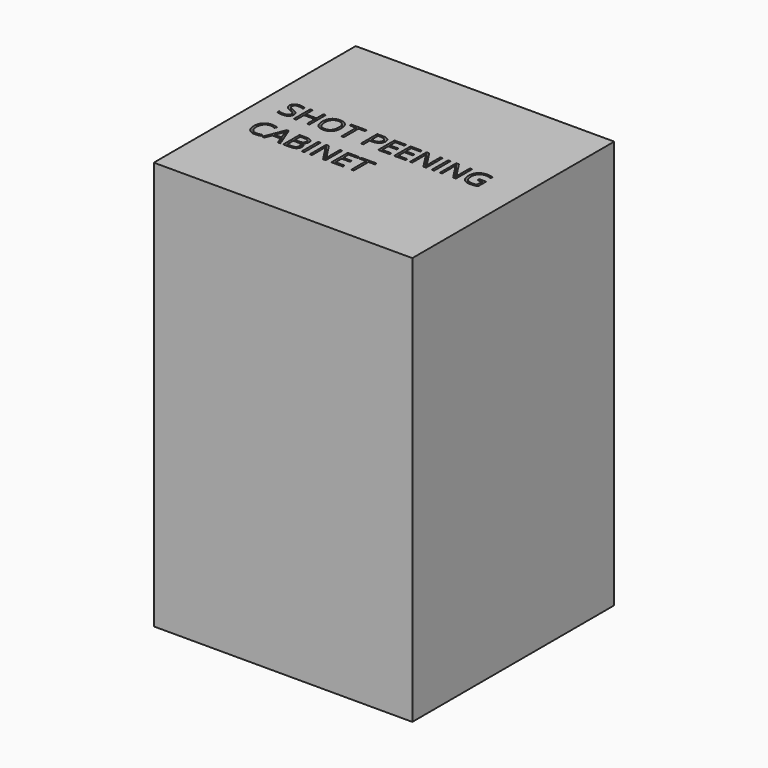
from build123d import *

# Parameters (mm, degrees)
F0_W         = 1260
F0_H         = 1230
F1_DEPTH     = 1990
F2_TEXT_SIZE = 140.1112564978
F3_DEPTH     = 1500


# Not quite as in the source:
# - Text() gives the source's letters only with a copy of the font that has no kerning and outlines rounded to 1/6400 em; it was checked with that copy


with BuildPart() as f1:
    # F0 (on Top) → F1 (new body)
    with BuildSketch(Plane.XY):
        Rectangle(F0_W, F0_H)
    extrude(amount=F1_DEPTH)

    # F2 (on face) → F3 (cut)
    with BuildSketch(Plane.XY.offset(1990)):
        with Locations((-530, 0)):
            Text('SHOT PEENING', F2_TEXT_SIZE, font='Open Sans', text_align=(TextAlign.LEFT, TextAlign.BOTTOM))
        with Locations((-530, -190.5513088369)):
            Text('CABINET', F2_TEXT_SIZE, font='Open Sans', text_align=(TextAlign.LEFT, TextAlign.BOTTOM))
    extrude(amount=-F3_DEPTH, mode=Mode.SUBTRACT)


solid = f1.part
